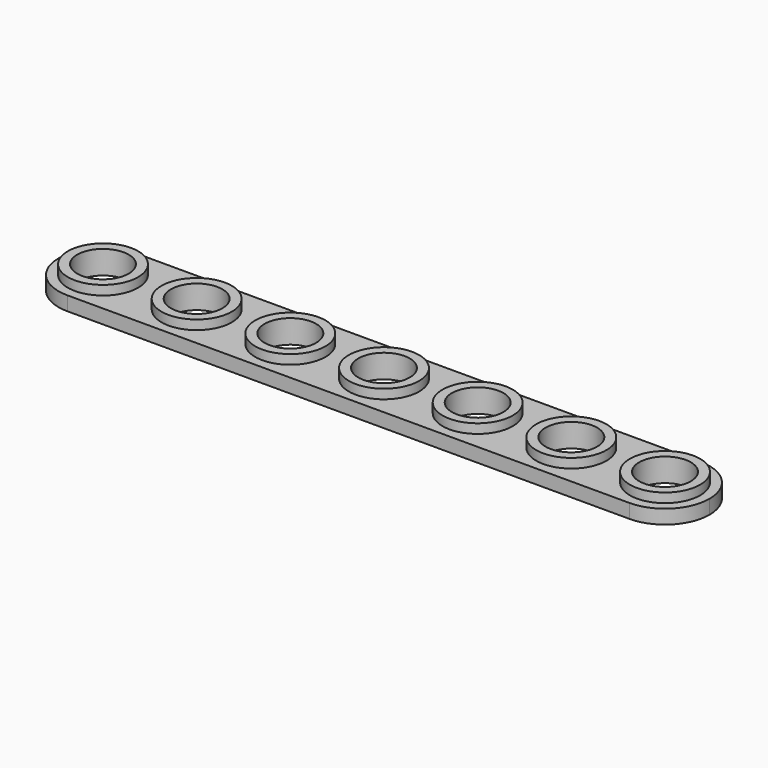
from build123d import *

# Parameters (mm, degrees)
F2_R     = 7.5
F2_R_2   = 5.5
F3_DEPTH = 3
F4_DEPTH = 5


# Not quite as in the source:
# - a feature names something its author has since deleted; it is built from what else it names


with BuildPart() as f3:
    # F2 (on Top) → F3 (new body)
    with BuildSketch(Plane.XY):
        with BuildLine():
            Line((120, 9.5), (0, 9.5))
            ThreePointArc((0, 9.5), (-6.7175144213, 6.7175144213), (-9.5, 0))
            ThreePointArc((-9.5, 0), (-6.7175144213, -6.7175144213), (0, -9.5))
            Line((0, -9.5), (120, -9.5))
            ThreePointArc((120, -9.5), (126.7175144213, -6.7175144213), (129.5, 0))
            ThreePointArc((129.5, 0), (126.7175144213, 6.7175144213), (120, 9.5))
        make_face()
        Circle(F2_R, mode=Mode.SUBTRACT)
        with Locations((20, 0)):
            Circle(F2_R, mode=Mode.SUBTRACT)
        with Locations((40, 0)):
            Circle(F2_R, mode=Mode.SUBTRACT)
        with Locations((60, 0)):
            Circle(F2_R, mode=Mode.SUBTRACT)
        with Locations((80, 0)):
            Circle(F2_R, mode=Mode.SUBTRACT)
        with Locations((100, 0)):
            Circle(F2_R, mode=Mode.SUBTRACT)
        with Locations((120, 0)):
            Circle(F2_R, mode=Mode.SUBTRACT)
        Circle(F2_R)
        Circle(F2_R_2, mode=Mode.SUBTRACT)
        with Locations((20, 0)):
            Circle(F2_R)
        with Locations((20, 0)):
            Circle(F2_R_2, mode=Mode.SUBTRACT)
        with Locations((40, 0)):
            Circle(F2_R)
        with Locations((40, 0)):
            Circle(F2_R_2, mode=Mode.SUBTRACT)
        with Locations((60, 0)):
            Circle(F2_R)
        with Locations((60, 0)):
            Circle(F2_R_2, mode=Mode.SUBTRACT)
        with Locations((80, 0)):
            Circle(F2_R)
        with Locations((80, 0)):
            Circle(F2_R_2, mode=Mode.SUBTRACT)
        with Locations((100, 0)):
            Circle(F2_R)
        with Locations((100, 0)):
            Circle(F2_R_2, mode=Mode.SUBTRACT)
        with Locations((120, 0)):
            Circle(F2_R)
        with Locations((120, 0)):
            Circle(F2_R_2, mode=Mode.SUBTRACT)
    extrude(amount=F3_DEPTH)

    # F2 (on Top) → F4 (join)
    with BuildSketch(Plane.XY):
        Circle(F2_R)
        Circle(F2_R_2, mode=Mode.SUBTRACT)
        with Locations((20, 0)):
            Circle(F2_R)
        with Locations((20, 0)):
            Circle(F2_R_2, mode=Mode.SUBTRACT)
        with Locations((40, 0)):
            Circle(F2_R)
        with Locations((40, 0)):
            Circle(F2_R_2, mode=Mode.SUBTRACT)
        with Locations((60, 0)):
            Circle(F2_R)
        with Locations((60, 0)):
            Circle(F2_R_2, mode=Mode.SUBTRACT)
        with Locations((80, 0)):
            Circle(F2_R)
        with Locations((80, 0)):
            Circle(F2_R_2, mode=Mode.SUBTRACT)
        with Locations((100, 0)):
            Circle(F2_R)
        with Locations((100, 0)):
            Circle(F2_R_2, mode=Mode.SUBTRACT)
        with Locations((120, 0)):
            Circle(F2_R)
        with Locations((120, 0)):
            Circle(F2_R_2, mode=Mode.SUBTRACT)
    extrude(amount=F4_DEPTH)


solid = f3.part
